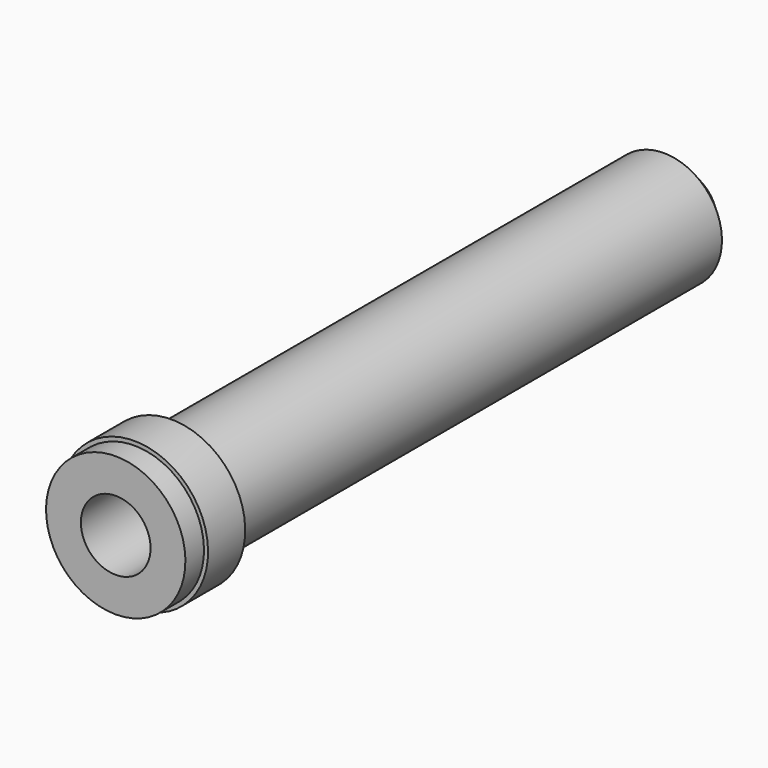
from build123d import *

# Parameters (mm, degrees)
F3_SIZE2 = 2
F3_SIZE  = 2


# Not quite as in the source:
# - a feature names something its author has since deleted; it is built from what else it names


with BuildPart() as f1:
    # F0 (on Right) → F1 (revolve)
    with BuildSketch(Plane.YZ):
        Polygon((-7.8531129844, -6), (-5.8531129844, -6), (-5.8531129844, -6.35), (-1.8531129844, -6.35), (-1.8531129844, -5), (45.1962463558, -5), (53.1468870156, -5), (53.1468870156, 0), (7.1468870156, 0), (5, -3), (-7.8531129844, -3), (-7.8531129844, -5.5), align=None)
    revolve(axis=Axis((0, 30.1468870156, 0), (0, -1, 0)))

    # F3
    f3_edges = [f1.edges().sort_by_distance(p)[0] for p in [
        (0, 53.146887, 5),
    ]]
    chamfer(f3_edges, length=F3_SIZE, length2=F3_SIZE2)


solid = f1.part
